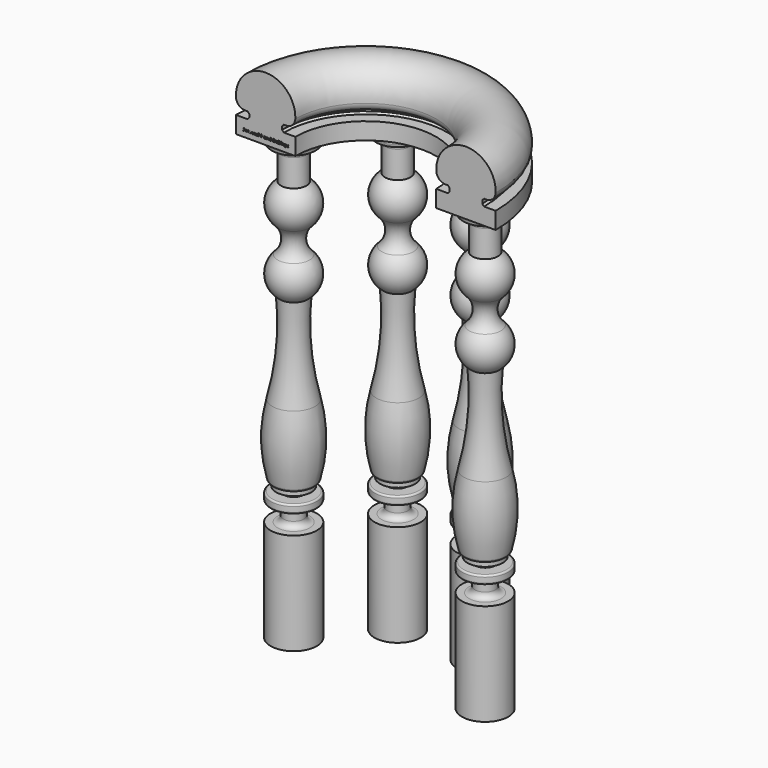
from build123d import *

# Parameters (mm, degrees)
F1_ANGLE     = 180
F6_R         = 2.286
F8_COUNT     = 4
F8_ANGLE     = 145.6939
F9_TEXT_SIZE = 5.5799648506
F10_DEPTH    = 0.635


# Not quite as in the source:
# - Text() gives the source's letters only with a copy of the font that has no kerning and outlines rounded to 1/6400 em; it was checked with that copy


with BuildPart() as f1:
    # F0 (on Front) → F1 (revolve)
    with BuildSketch(Plane.XZ):
        with BuildLine():
            ThreePointArc((-40.7305715834, -1.9298005112), (-36.8099805199, -10.5190551207), (-28.0448023112, -14.0287531142))
            Line((-28.0448023112, -14.0287531142), (-24.950685116, -14.0287531142))
            Line((-24.950685116, -14.0287531142), (-22.4087256938, -16.5707125364))
            Line((-22.4087256938, -16.5707125364), (-22.4087256938, -21.0157125364))
            Line((-22.4087256938, -21.0157125364), (-24.950685116, -23.5576719585))
            Line((-24.950685116, -23.5576719585), (-40.7762625988, -23.5576719585))
            Line((-40.7762625988, -23.5576719585), (-40.7762625988, -46.8012571457))
            Line((-40.7762625988, -46.8012571457), (40.7762625988, -46.8012571457))
            Line((40.7762625988, -46.8012571457), (40.7762625988, -23.5576719585))
            Line((40.7762625988, -23.5576719585), (24.950685116, -23.5576719585))
            Line((24.950685116, -23.5576719585), (22.4087256938, -21.0157125364))
            Line((22.4087256938, -21.0157125364), (22.4087256938, -16.5707125364))
            Line((22.4087256938, -16.5707125364), (24.950685116, -14.0287531142))
            Line((24.950685116, -14.0287531142), (28.0448023112, -14.0287531142))
            ThreePointArc((28.0448023112, -14.0287531142), (36.8099805199, -10.5190551207), (40.7305715834, -1.9298005112))
            ThreePointArc((40.7305715834, -1.9298005112), (0, 40.7762625988), (-40.7305715834, -1.9298005112))
        make_face()
    revolve(axis=Axis((137.4897807837, 0, -15.0512571457), (0, 0, -1)), revolution_arc=F1_ANGLE)

    # F9 (on Front) → F10 (cut)
    with BuildSketch(Plane.XZ):
        with Locations((-31.75, -39.5737321632)):
            Text('Berrocal Hand-Railings', F9_TEXT_SIZE, font='Open Sans', font_style=FontStyle.BOLD, text_align=(TextAlign.LEFT, TextAlign.BOTTOM))
    extrude(amount=-F10_DEPTH, mode=Mode.SUBTRACT)


with BuildPart() as f5:
    # F4 (on plane+point) → F5 (revolve)
    with BuildSketch(Plane.XZ.offset(-40.54931088)):
        with BuildLine():
            Line((6.1155321384, -342.5117463768), (6.1155321384, -656.4012571457))
            Line((6.1155321384, -656.4012571457), (37.8655321384, -656.4012571457))
            Line((37.8655321384, -656.4012571457), (37.8655321384, -516.7012571457))
            Line((37.8655321384, -516.7012571457), (28.1659383513, -516.7012571457))
            ThreePointArc((28.1659383513, -516.7012571457), (22.5063462375, -514.3569773347), (20.1620664265, -508.6973852209))
            Line((20.1620664265, -508.6973852209), (20.1620664265, -490.958078211))
            Line((20.1620664265, -490.958078211), (37.8655321384, -490.958078211))
            Line((37.8655321384, -490.958078211), (37.8655321384, -479.3219664687))
            Line((37.8655321384, -479.3219664687), (20.1620664265, -479.3219664687))
            Line((20.1620664265, -479.3219664687), (20.1620664265, -472.9719664687))
            Line((20.1620664265, -472.9719664687), (30.2455321384, -472.9719664687))
            Line((30.2455321384, -472.9719664687), (30.2455321384, -466.6219664687))
            ThreePointArc((30.2455321384, -466.6219664687), (33.1923159868, -465.6178430956), (34.9128526169, -463.023319536))
            ThreePointArc((34.9128526169, -463.023319536), (41.1748672542, -415.3682102704), (35.3098359688, -367.6626165266))
            ThreePointArc((35.3098359688, -367.6626165266), (24.9481261953, -305.0638110724), (25.2986469452, -241.6142042264))
            ThreePointArc((25.2986469452, -241.6142042264), (37.8205911901, -218.0032942675), (27.8775550205, -193.1958319127))
            ThreePointArc((27.8775550205, -193.1958319127), (19.4846427223, -173.769106578), (27.8775550205, -154.3423812434))
            ThreePointArc((27.8775550205, -154.3423812434), (37.747081211, -128.4836250559), (23.5780321384, -104.7071478743))
            Line((23.5780321384, -104.7071478743), (23.5780321384, -67.5051290705))
            ThreePointArc((23.5780321384, -67.5051290705), (25.9223119495, -61.8455369567), (31.5819040633, -59.5012571457))
            Line((31.5819040633, -59.5012571457), (32.7855321384, -59.5012571457))
            ThreePointArc((32.7855321384, -59.5012571457), (36.3776345869, -58.0133595941), (37.8655321384, -54.4212571457))
            Line((37.8655321384, -54.4212571457), (37.8655321384, -51.8812571457))
            ThreePointArc((37.8655321384, -51.8812571457), (36.3776345869, -48.2891546973), (32.7855321384, -46.8012571457))
            Line((32.7855321384, -46.8012571457), (24.7690393744, -46.8012571457))
            Line((24.7690393744, -46.8012571457), (6.1155321384, -46.8012571457))
            Line((6.1155321384, -46.8012571457), (6.1155321384, -172.2432451062))
            Line((6.1155321384, -172.2432451062), (6.1155321384, -223.8556616873))
            Line((6.1155321384, -223.8556616873), (6.1155321384, -342.5117463768))
        make_face()
    revolve(axis=Axis((6.1155321384, 40.54931088, -688.8244650902), (0, 0, -1)))

    # F6
    f6_edges = [f5.edges().sort_by_distance(p)[0] for p in [
        (-7.931002, 40.549311, -508.697385),
        (-7.931002, 40.549311, -490.958078),
        (20.162066, 40.549311, -499.827732),
        (-25.634468, 40.549311, -490.958078),
        (-25.634468, 40.549311, -479.321966),
    ]]
    fillet(f6_edges, radius=F6_R)


with BuildPart() as f8_1:
    # F8: instance of F5
    add(f5.part.rotate(Axis((137.4897807837, 0, 20.3341305195), (0, 0, -1)), 1 * F8_ANGLE / (F8_COUNT - 1)))


with BuildPart() as f8_2:
    # F8: instance of F5
    add(f5.part.rotate(Axis((137.4897807837, 0, 20.3341305195), (0, 0, -1)), 2 * F8_ANGLE / (F8_COUNT - 1)))


with BuildPart() as f8_3:
    # F8: instance of F5
    add(f5.part.rotate(Axis((137.4897807837, 0, 20.3341305195), (0, 0, -1)), 3 * F8_ANGLE / (F8_COUNT - 1)))


solid = Compound([f1.part, f5.part, f8_1.part, f8_2.part, f8_3.part])
